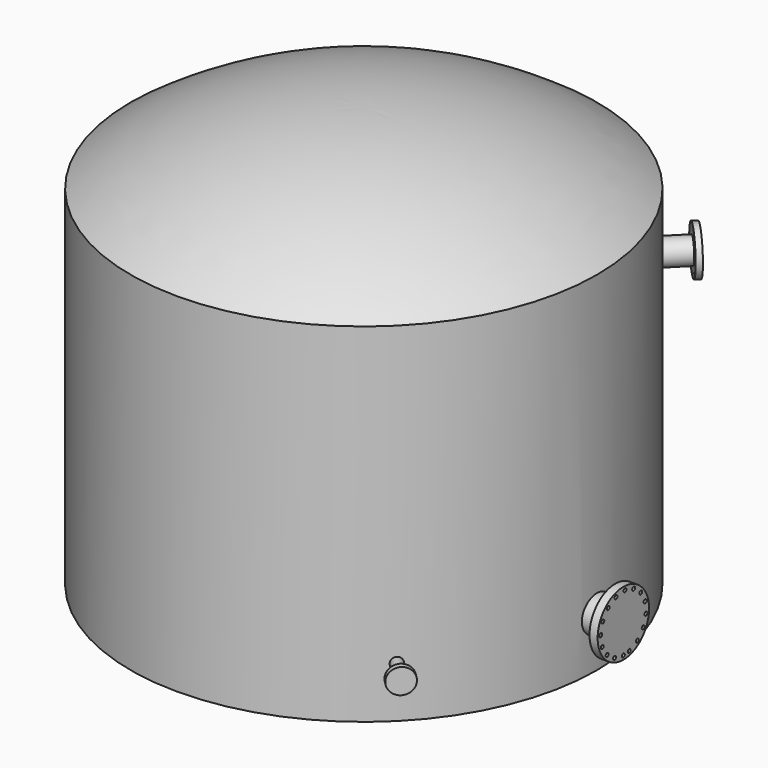
from build123d import *

# Parameters (mm, degrees)
F3_R      = 80
F4_DEPTH  = 80
F5_R      = 142
F6_DEPTH  = 36
F7_R      = 8
F8_DEPTH  = 75
F10_R     = 55
F11_DEPTH = 110
F12_R     = 102
F13_DEPTH = 25
F14_R     = 6
F15_DEPTH = 75
F18_R     = 55
F19_DEPTH = 110
F20_R     = 102
F21_DEPTH = 25
F22_R     = 6
F23_DEPTH = 75
F26_R     = 25
F27_DEPTH = 110
F28_R     = 55
F29_DEPTH = 25


with BuildPart() as f1:
    # F0 (on Front) → F1 (revolve)
    with BuildSketch(Plane.XZ):
        with BuildLine():
            Line((0, 1741.8010112751), (0, -113.1989887249))
            Line((0, -113.1989887249), (1030, -113.1989887249))
            Line((1030, -113.1989887249), (1030, 1423.8010112751))
            ThreePointArc((1030, 1423.8010112751), (540.2165034856, 1664.4771074705), (0, 1741.8010112751))
        make_face()
    revolve(axis=Axis((0, 0, -221.1202199703), (0, 0, 1)))

    # F3 (on offset) → F4 (join, symmetric)
    with BuildSketch(Plane.YZ.offset(1030)):
        with Locations((0, 106.8010112751)):
            Circle(F3_R)
    extrude(amount=F4_DEPTH, both=True)

    # F5 (on face) → F6 (join)
    with BuildSketch(Plane.YZ.offset(1110)):
        with Locations((0, 106.8010112751)):
            Circle(F5_R)
    extrude(amount=F6_DEPTH)

    # F7 (on face) → F8 (cut)
    with BuildSketch(Plane.YZ.offset(1146)):
        with Locations((0, -18.1989887249)):
            Circle(F7_R)
        with Locations((-48.8413910612, -8.2620954065)):
            Circle(F7_R)
        with Locations((-89.9174750423, 19.9687149677)):
            Circle(F7_R)
        with Locations((-116.6975533122, 62.0050175819)):
            Circle(F7_R)
        with Locations((-124.9238533774, 111.1634483629)):
            Circle(F7_R)
        with Locations((-113.2884733796, 159.6282939927)):
            Circle(F7_R)
        with Locations((-83.6413257949, 199.6941144598)):
            Circle(F7_R)
        with Locations((-40.6960193071, 224.990833225)):
            Circle(F7_R)
        with Locations((8.719559218, 231.4965175576)):
            Circle(F7_R)
        with Locations((56.7488124674, 218.1768267986)):
            Circle(F7_R)
        with Locations((95.7555553899, 187.1494624859)):
            Circle(F7_R)
        with Locations((119.5380944954, 143.3474743654)):
            Circle(F7_R)
        with Locations((124.315236921, 93.7349533666)):
            Circle(F7_R)
        with Locations((109.3274633924, 46.1998087443)):
            Circle(F7_R)
        with Locations((76.9576844157, 8.2996670743)):
            Circle(F7_R)
        with Locations((32.3523806378, -13.939717011)):
            Circle(F7_R)
    extrude(amount=-F8_DEPTH, mode=Mode.SUBTRACT)


with BuildPart() as f11:
    # F10 (on offset) → F11 (new body)
    with BuildSketch(Plane.YZ.offset(-1030)):
        with Locations((0, 1118.8010112751)):
            Circle(F10_R)
    extrude(amount=-F11_DEPTH)

    # F12 (on face) → F13 (join)
    with BuildSketch(Plane(origin=(-1140, 0, 0), x_dir=(0, -1, 0), z_dir=(-1, 0, 0))):
        with Locations((0, 1118.8010112751)):
            Circle(F12_R)
    extrude(amount=F13_DEPTH)

    # F14 (on face) → F15 (cut)
    with BuildSketch(Plane(origin=(-1165, 0, 0), x_dir=(0, -1, 0), z_dir=(-1, 0, 0))):
        with Locations((0, 1199.8010112751)):
            Circle(F14_R)
        with Locations((-1039.0581552505, -599.9005056375)):
            Circle(F14_R)
        with Locations((1039.0581552505, -599.9005056376)):
            Circle(F14_R)
        with Locations((63.3283500799, 1169.3036852257)):
            Circle(F14_R)
        with Locations((78.9691608867, 1100.7768156246)):
            Circle(F14_R)
        with Locations((35.1445828685, 1045.822532975)):
            Circle(F14_R)
        with Locations((-35.1445828685, 1045.822532975)):
            Circle(F14_R)
        with Locations((-78.9691608867, 1100.7768156246)):
            Circle(F14_R)
        with Locations((-63.3283500799, 1169.3036852257)):
            Circle(F14_R)
    extrude(amount=-F15_DEPTH, mode=Mode.SUBTRACT)


with BuildPart() as f19:
    # F18 (on face) → F19 (new body)
    with BuildSketch(Plane(origin=(728.3199846221, 728.3199846221, 0), x_dir=(-0.7071067812, 0.7071067812, 0), z_dir=(0.7071067812, 0.7071067812, 0))):
        with Locations((0, 1118.8010112751)):
            Circle(F18_R)
    extrude(amount=F19_DEPTH)

    # F20 (on face) → F21 (join)
    with BuildSketch(Plane(origin=(806.1017305527, 806.1017305527, 0), x_dir=(-0.7071067812, 0.7071067812, 0), z_dir=(0.7071067812, 0.7071067812, 0))):
        with Locations((0, 1118.8010112751)):
            Circle(F20_R)
    extrude(amount=F21_DEPTH)

    # F22 (on face) → F23 (cut)
    with BuildSketch(Plane(origin=(823.7794000823, 823.7794000823, 0), x_dir=(-0.7071067812, 0.7071067812, 0), z_dir=(0.7071067812, 0.7071067812, 0))):
        with Locations((0, 1205.8010112751)):
            Circle(F22_R)
        with Locations((-61.5182899632, 1180.3193012383)):
            Circle(F22_R)
        with Locations((-87, 1118.8010112751)):
            Circle(F22_R)
        with Locations((-61.5182899632, 1057.2827213119)):
            Circle(F22_R)
        with Locations((0, 1031.8010112751)):
            Circle(F22_R)
        with Locations((61.5182899632, 1057.2827213119)):
            Circle(F22_R)
        with Locations((87, 1118.8010112751)):
            Circle(F22_R)
        with Locations((61.5182899632, 1180.3193012383)):
            Circle(F22_R)
    extrude(amount=-F23_DEPTH, mode=Mode.SUBTRACT)


with BuildPart() as f27:
    # F26 (on face) → F27 (new body)
    with BuildSketch(Plane(origin=(728.3199846221, -728.3199846221, 0), x_dir=(-0.7071067812, -0.7071067812, 0), z_dir=(-0.7071067812, 0.7071067812, 0))):
        with Locations((0, 111.8010112751)):
            Circle(F26_R)
    extrude(amount=-F27_DEPTH)

    # F28 (on face) → F29 (join)
    with BuildSketch(Plane(origin=(806.1017305527, -806.1017305527, 0), x_dir=(0.7071067812, 0.7071067812, 0), z_dir=(0.7071067812, -0.7071067812, 0))):
        with Locations((0, 111.8010112751)):
            Circle(F28_R)
    extrude(amount=F29_DEPTH)


solid = Compound([f1.part, f11.part, f19.part, f27.part])
